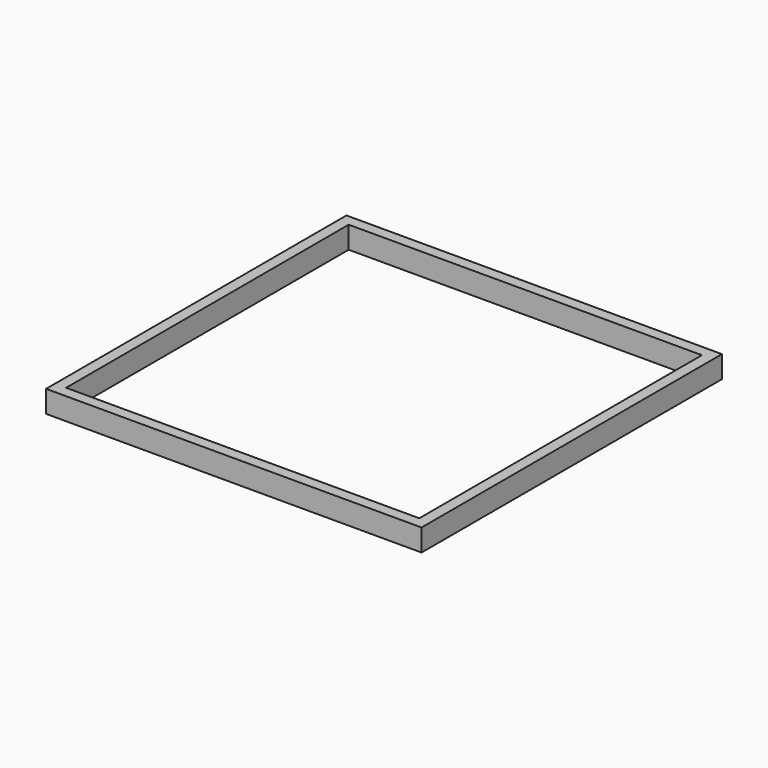
from build123d import *

# Parameters (mm, degrees)
F0_W     = 270
F0_H     = 270
F0_W_2   = 254
F0_H_2   = 254
F1_DEPTH = 15.875


# Not quite as in the source:
# - a length typed as a fraction of an inch, garbled in the dataset ("3 / 203.2 mm" for 3/8 in), is restored


with BuildPart() as f1:
    # F0 (on Top) → F1 (new body)
    with BuildSketch(Plane.XY):
        Rectangle(F0_W, F0_H)
        Rectangle(F0_W_2, F0_H_2, mode=Mode.SUBTRACT)
    extrude(amount=F1_DEPTH)


solid = f1.part
